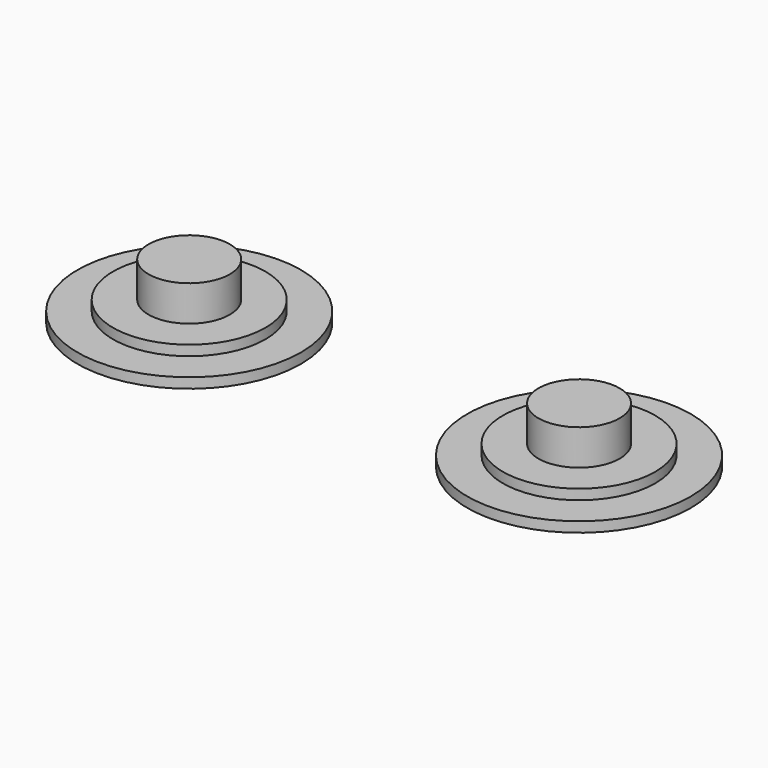
from build123d import *

# Parameters (mm, degrees)
F0_R     = 11
F0_R_2   = 7.5
F1_DEPTH = 1
F0_R_3   = 4
F2_DEPTH = 2
F3_DEPTH = 5.5


with BuildPart() as f1:
    # F0 (on Top) → F1 (new body)
    with BuildSketch(Plane.XY):
        Circle(F0_R)
        Circle(F0_R_2, mode=Mode.SUBTRACT)
    extrude(amount=F1_DEPTH)

    # F0 (on Top) → F2 (join)
    with BuildSketch(Plane.XY):
        Circle(F0_R_2)
        Circle(F0_R_3, mode=Mode.SUBTRACT)
    extrude(amount=F2_DEPTH)

    # F0 (on Top) → F3 (join)
    with BuildSketch(Plane.XY):
        Circle(F0_R_3)
    extrude(amount=F3_DEPTH)


with BuildPart() as f1b:
    # F0 (on Top) → F1, piece 2 (new body)
    with BuildSketch(Plane.XY):
        with Locations((38.3674800396, 0)):
            Circle(F0_R)
        with Locations((38.3674800396, 0)):
            Circle(F0_R_2, mode=Mode.SUBTRACT)
    extrude(amount=F1_DEPTH)


with BuildPart() as f2:
    # F0 (on Top) → F2, piece 2 (new body)
    with BuildSketch(Plane.XY):
        with Locations((38.3674800396, 0)):
            Circle(F0_R_2)
        with Locations((38.3674800396, 0)):
            Circle(F0_R_3, mode=Mode.SUBTRACT)
    extrude(amount=F2_DEPTH)


with BuildPart() as f3:
    # F0 (on Top) → F3, piece 2 (new body)
    with BuildSketch(Plane.XY):
        with Locations((38.3674800396, 0)):
            Circle(F0_R_3)
    extrude(amount=F3_DEPTH)


solid = Compound([f1.part, f1b.part, f2.part, f3.part])
